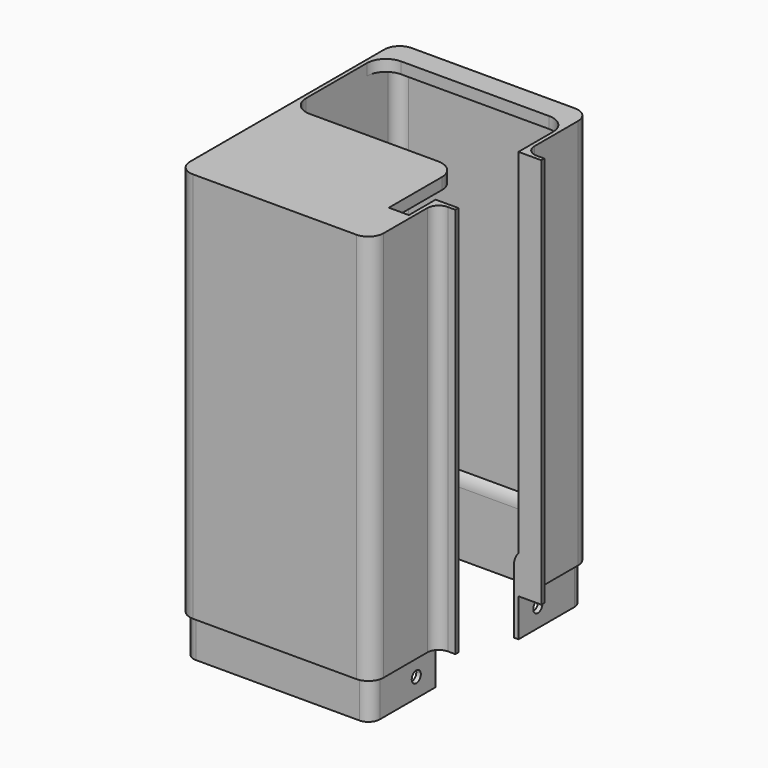
from build123d import *

# Parameters (mm, degrees)
F1_DEPTH     = 100
F3_DEPTH     = 3
F5_DEPTH     = 10
F6_R         = 1.5
F7_DEPTH     = 55.001
F8_T1_DEPTH  = 26.4990384046
F8_T3_DEPTH  = 43
F8_T5_DEPTH  = 64
F8_T7_DEPTH  = 26.4990384046
F8_T10_ANGLE = 90
F8_T12_ANGLE = 90
F8_T14_ANGLE = 90
F8_T16_ANGLE = 90
F9_W         = 5.2690437883
F9_H         = 22.4438142031
F10_DEPTH    = 25
F11_DEPTH    = 22.3
F12_R        = 5


# Not quite as in the source:
# - a fillet or chamfer that OpenCascade refuses, or shapes differently, is made with other operations: its cross-section is extruded or revolved along the edge and cut away or added
# - two fillets or chamfers of one size are made in one step


with BuildPart() as f1:
    # F0 (on Top) → F1 (new body)
    with BuildSketch(Plane.XY):
        with BuildLine():
            Line((-21.5, 35), (21.5, 35))
            ThreePointArc((21.5, 35), (23.6213203436, 34.1213203436), (24.5, 32))
            Line((24.5, 32), (24.5, 13.625))
            Line((24.5, 13.625), (30.5, 13.625))
            Line((30.5, 13.625), (30.5, 14.625))
            Line((30.5, 14.625), (28.5, 14.625))
            ThreePointArc((28.5, 14.625), (26.3786796564, 15.5036796564), (25.5, 17.625))
            Line((25.5, 17.625), (25.5, 32))
            ThreePointArc((25.5, 32), (24.3284271247, 34.8284271247), (21.5, 36))
            Line((21.5, 36), (-21.5, 36))
            ThreePointArc((-21.5, 36), (-24.3284271247, 34.8284271247), (-25.5, 32))
            Line((-25.5, 32), (-25.5, -32))
            ThreePointArc((-25.5, -32), (-24.3284271247, -34.8284271247), (-21.5, -36))
            Line((-21.5, -36), (21.5, -36))
            ThreePointArc((21.5, -36), (24.3284271247, -34.8284271247), (25.5, -32))
            Line((25.5, -32), (25.5, -17.625))
            ThreePointArc((25.5, -17.625), (26.3786796564, -15.5036796564), (28.5, -14.625))
            Line((28.5, -14.625), (30.5, -14.625))
            Line((30.5, -14.625), (30.5, -13.625))
            Line((30.5, -13.625), (24.5, -13.625))
            Line((24.5, -13.625), (24.5, -32))
            ThreePointArc((24.5, -32), (23.6213203436, -34.1213203436), (21.5, -35))
            Line((21.5, -35), (-21.5, -35))
            ThreePointArc((-21.5, -35), (-23.6213203436, -34.1213203436), (-24.5, -32))
            Line((-24.5, -32), (-24.5, 32))
            ThreePointArc((-24.5, 32), (-23.6213203436, 34.1213203436), (-21.5, 35))
        make_face()
    extrude(amount=F1_DEPTH)

    # F2 (on face) → F3 (join)
    with BuildSketch(Plane.XY.offset(100)):
        with BuildLine():
            Line((24.5, -32), (24.5, -13.625))
            Line((24.5, -13.625), (24.5, 0))
            Line((24.5, 0), (-24.5, 0))
            Line((-24.5, 0), (-24.5, -32))
            ThreePointArc((-24.5, -32), (-23.6213203436, -34.1213203436), (-21.5, -35))
            Line((-21.5, -35), (21.5, -35))
            ThreePointArc((21.5, -35), (23.6213203436, -34.1213203436), (24.5, -32))
        make_face()
        with BuildLine():
            Line((30.5, -13.625), (24.5, -13.625))
            Line((24.5, -13.625), (24.5, -32))
            ThreePointArc((24.5, -32), (23.6213203436, -34.1213203436), (21.5, -35))
            Line((21.5, -35), (-21.5, -35))
            ThreePointArc((-21.5, -35), (-23.6213203436, -34.1213203436), (-24.5, -32))
            Line((-24.5, -32), (-24.5, 0))
            Line((-24.5, 0), (-24.5, 30))
            Line((-24.5, 30), (-24.5, 32))
            ThreePointArc((-24.5, 32), (-23.6213203436, 34.1213203436), (-21.5, 35))
            Line((-21.5, 35), (21.5, 35))
            ThreePointArc((21.5, 35), (23.6213203436, 34.1213203436), (24.5, 32))
            Line((24.5, 32), (24.5, 30))
            Line((24.5, 30), (24.5, 13.625))
            Line((24.5, 13.625), (30.5, 13.625))
            Line((30.5, 13.625), (30.5, 14.625))
            Line((30.5, 14.625), (28.5, 14.625))
            ThreePointArc((28.5, 14.625), (26.3786796564, 15.5036796564), (25.5, 17.625))
            Line((25.5, 17.625), (25.5, 32))
            ThreePointArc((25.5, 32), (24.3284271247, 34.8284271247), (21.5, 36))
            Line((21.5, 36), (-21.5, 36))
            ThreePointArc((-21.5, 36), (-24.3284271247, 34.8284271247), (-25.5, 32))
            Line((-25.5, 32), (-25.5, -32))
            ThreePointArc((-25.5, -32), (-24.3284271247, -34.8284271247), (-21.5, -36))
            Line((-21.5, -36), (21.5, -36))
            ThreePointArc((21.5, -36), (24.3284271247, -34.8284271247), (25.5, -32))
            Line((25.5, -32), (25.5, -17.625))
            ThreePointArc((25.5, -17.625), (26.3786796564, -15.5036796564), (28.5, -14.625))
            Line((28.5, -14.625), (30.5, -14.625))
            Line((30.5, -14.625), (30.5, -13.625))
        make_face()
        with BuildLine():
            Line((-24.5, 32), (-24.5, 30))
            Line((-24.5, 30), (24.5, 30))
            Line((24.5, 30), (24.5, 32))
            ThreePointArc((24.5, 32), (23.6213203436, 34.1213203436), (21.5, 35))
            Line((21.5, 35), (-21.5, 35))
            ThreePointArc((-21.5, 35), (-23.6213203436, 34.1213203436), (-24.5, 32))
        make_face()
    extrude(amount=F3_DEPTH)

    # F4 (on face) → F5 (join, symmetric)
    with BuildSketch(Plane(origin=(0, 0, 0), x_dir=(1, 0, 0), z_dir=(0, 0, -1))):
        with BuildLine():
            Line((23.3, -13.625), (23.3, -32))
            ThreePointArc((23.3, -32), (22.7727922061, -33.2727922061), (21.5, -33.8))
            Line((21.5, -33.8), (-21.5, -33.8))
            ThreePointArc((-21.5, -33.8), (-22.7727922061, -33.2727922061), (-23.3, -32))
            Line((-23.3, -32), (-23.3, 32))
            ThreePointArc((-23.3, 32), (-22.7727922061, 33.2727922061), (-21.5, 33.8))
            Line((-21.5, 33.8), (21.5, 33.8))
            ThreePointArc((21.5, 33.8), (22.7727922061, 33.2727922061), (23.3, 32))
            Line((23.3, 32), (23.3, 13.625))
            Line((23.3, 13.625), (24.5, 13.625))
            Line((24.5, 13.625), (24.5, 32))
            ThreePointArc((24.5, 32), (23.6213203436, 34.1213203436), (21.5, 35))
            Line((21.5, 35), (-21.5, 35))
            ThreePointArc((-21.5, 35), (-23.6213203436, 34.1213203436), (-24.5, 32))
            Line((-24.5, 32), (-24.5, -32))
            ThreePointArc((-24.5, -32), (-23.6213203436, -34.1213203436), (-21.5, -35))
            Line((-21.5, -35), (21.5, -35))
            ThreePointArc((21.5, -35), (23.6213203436, -34.1213203436), (24.5, -32))
            Line((24.5, -32), (24.5, -13.625))
            Line((24.5, -13.625), (23.3, -13.625))
        make_face()
    extrude(amount=F5_DEPTH, both=True)

    # F6 (on face) → F7 (cut, through all)
    with BuildSketch(Plane(origin=(-24.5, 0, 0), x_dir=(0, -1, 0), z_dir=(-1, 0, 0))):
        with Locations((-20, -5)):
            Circle(F6_R)
        with Locations((20, -5)):
            Circle(F6_R)
    extrude(amount=-F7_DEPTH, mode=Mode.SUBTRACT)

    # F8: fillet of radius 5 on 1 edges, made by hand

    # F8_s2 → F8_t1 (cut)
    with BuildSketch(Plane.XZ.offset(-32)):
        with BuildLine():
            ThreePointArc((24.5, 10), (23.6095842402, 8.4824354457), (23.3, 6.7503846381))
            Line((23.3, 6.7503846381), (23.3, 10))
            Line((23.3, 10), (24.5, 10))
        make_face()
    extrude(amount=F8_T1_DEPTH, mode=Mode.SUBTRACT)

    # F8_s4 → F8_t3 (cut)
    with BuildSketch(Plane.YZ.offset(-21.5)):
        with BuildLine():
            ThreePointArc((35, 10), (34.1095842402, 8.4824354457), (33.8, 6.7503846381))
            Line((33.8, 6.7503846381), (33.8, 10))
            Line((33.8, 10), (35, 10))
        make_face()
        with BuildLine():
            ThreePointArc((-35, 10), (-34.1095842402, 8.4824354457), (-33.8, 6.7503846381))
            Line((-33.8, 6.7503846381), (-33.8, 10))
            Line((-33.8, 10), (-35, 10))
        make_face()
    extrude(amount=F8_T3_DEPTH, mode=Mode.SUBTRACT)

    # F8_s6 → F8_t5 (cut)
    with BuildSketch(Plane.XZ.offset(-32)):
        with BuildLine():
            ThreePointArc((-24.5, 10), (-23.6095842402, 8.4824354457), (-23.3, 6.7503846381))
            Line((-23.3, 6.7503846381), (-23.3, 10))
            Line((-23.3, 10), (-24.5, 10))
        make_face()
    extrude(amount=F8_T5_DEPTH, mode=Mode.SUBTRACT)

    # F8_s8 → F8_t7 (cut)
    with BuildSketch(Plane.XZ.offset(5.5009615954)):
        with BuildLine():
            ThreePointArc((24.5, 10), (23.6095842402, 8.4824354457), (23.3, 6.7503846381))
            Line((23.3, 6.7503846381), (23.3, 10))
            Line((23.3, 10), (24.5, 10))
        make_face()
    extrude(amount=F8_T7_DEPTH, mode=Mode.SUBTRACT)

    # F8_s9 → F8_t10 (revolve, cut)
    with BuildSketch(Plane.XZ.offset(-32)):
        with BuildLine():
            ThreePointArc((24.5, 10), (23.6095842402, 8.4824354457), (23.3, 6.7503846381))
            Line((23.3, 6.7503846381), (23.3, 10))
            Line((23.3, 10), (24.5, 10))
        make_face()
    revolve(axis=Axis((21.5, 32, 10), (0, 0, 1)), revolution_arc=F8_T10_ANGLE, mode=Mode.SUBTRACT)

    # F8_s11 → F8_t12 (revolve, cut)
    with BuildSketch(Plane.YZ.offset(-21.5)):
        with BuildLine():
            ThreePointArc((35, 10), (34.1095842402, 8.4824354457), (33.8, 6.7503846381))
            Line((33.8, 6.7503846381), (33.8, 10))
            Line((33.8, 10), (35, 10))
        make_face()
    revolve(axis=Axis((-21.5, 32, 10), (0, 0, 1)), revolution_arc=F8_T12_ANGLE, mode=Mode.SUBTRACT)

    # F8_s13 → F8_t14 (revolve, cut)
    with BuildSketch(Plane.XZ.offset(32)):
        with BuildLine():
            ThreePointArc((-24.5, 10), (-23.6095842402, 8.4824354457), (-23.3, 6.7503846381))
            Line((-23.3, 6.7503846381), (-23.3, 10))
            Line((-23.3, 10), (-24.5, 10))
        make_face()
    revolve(axis=Axis((-21.5, -32, 10), (0, 0, 1)), revolution_arc=F8_T14_ANGLE, mode=Mode.SUBTRACT)

    # F8_s15 → F8_t16 (revolve, cut)
    with BuildSketch(Plane.YZ.offset(21.5)):
        with BuildLine():
            ThreePointArc((-35, 10), (-34.1095842402, 8.4824354457), (-33.8, 6.7503846381))
            Line((-33.8, 6.7503846381), (-33.8, 10))
            Line((-33.8, 10), (-35, 10))
        make_face()
    revolve(axis=Axis((21.5, -32, 10), (0, 0, 1)), revolution_arc=F8_T16_ANGLE, mode=Mode.SUBTRACT)

    # F9 (on face) → F10 (cut)
    with BuildSketch(Plane.XY.offset(103)):
        with Locations((21.8654781058, -11.2219071016)):
            Rectangle(F9_W, F9_H)
    extrude(amount=-F10_DEPTH, mode=Mode.SUBTRACT)

    # F9 (on face) → F11 (cut)
    with BuildSketch(Plane.XY.offset(103)):
        Polygon((24.5, -13.625), (24.5, 0), (19.2309562117, 0), (19.2309562117, -22.4438142031), (24.5, -22.4438142031), align=None)
    extrude(amount=-F11_DEPTH, mode=Mode.SUBTRACT)

    # F12
    f12_edges = [f1.edges().sort_by_distance(p)[0] for p in [
        (-24.5, 0, 101.5),
        (19.230956, 0, 101.5),
        (-24.5, 30, 101.5),
        (24.5, 30, 101.5),
    ]]
    fillet(f12_edges, radius=F12_R)


solid = f1.part
